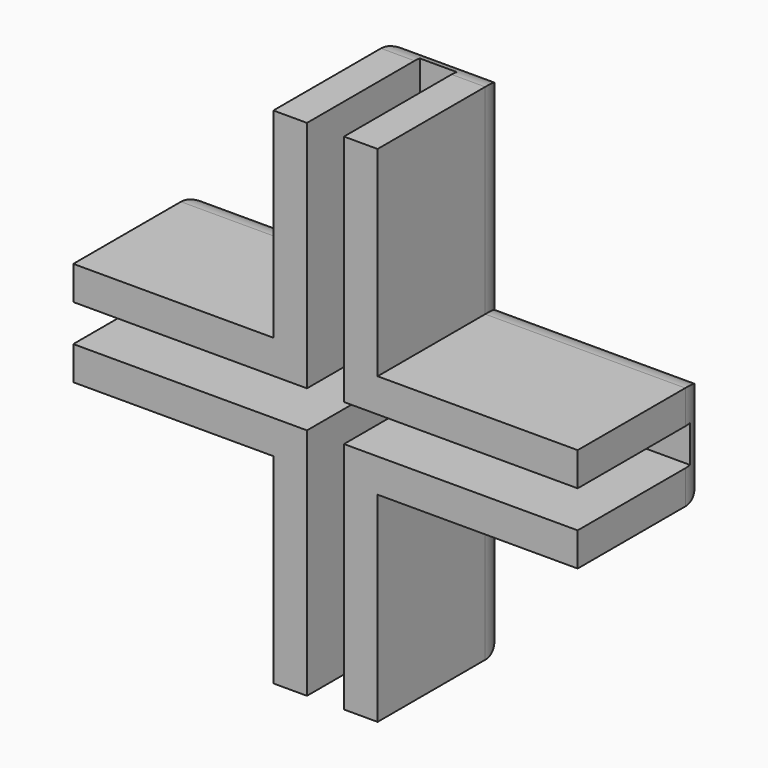
from build123d import *

# Parameters (mm, degrees)
F1_DEPTH     = 2.032
F2_DEPTH     = 12.7
F3_T1_DEPTH  = 21.463
F3_T3_DEPTH  = 21.463
F3_T5_DEPTH  = 20.574
F3_T7_DEPTH  = 21.463
F3_T9_DEPTH  = 20.574
F3_T11_DEPTH = 21.463
F3_T17_DEPTH = 27.813
F3_T21_DEPTH = 27.813
F3_T28_DEPTH = 27.813
F3_T32_DEPTH = 27.813
F3_T39_DEPTH = 27.813
F3_T43_DEPTH = 27.813
F3_T50_DEPTH = 27.813
F3_T54_DEPTH = 27.813


# Not quite as in the source:
# - a fillet or chamfer that OpenCascade refuses, or shapes differently, is made with other operations: its cross-section is extruded or revolved along the edge and cut away or added


with BuildPart() as f1:
    # F0 (on Front) → F1 (new body)
    with BuildSketch(Plane.XZ):
        Polygon((1.397, 19.05), (-1.397, 19.05), (-1.397, 1.397), (-19.05, 1.397), (-19.05, -1.397), (-1.397, -1.397), (-1.397, -19.05), (1.397, -19.05), (1.397, -1.397), (19.05, -1.397), (19.05, 1.397), (1.397, 1.397), align=None)
    extrude(amount=F1_DEPTH)

    # F0 (on Front) → F2 (join)
    with BuildSketch(Plane.XZ):
        Polygon((-1.397, 19.05), (-3.937, 19.05), (-3.937, 3.937), (-19.05, 3.937), (-19.05, 1.397), (-1.397, 1.397), align=None)
        Polygon((3.937, 19.05), (1.397, 19.05), (1.397, 1.397), (19.05, 1.397), (19.05, 3.937), (3.937, 3.937), align=None)
        Polygon((-1.397, -1.397), (-19.05, -1.397), (-19.05, -3.937), (-3.937, -3.937), (-3.937, -19.05), (-1.397, -19.05), align=None)
        Polygon((19.05, -3.937), (19.05, -1.397), (1.397, -1.397), (1.397, -19.05), (3.937, -19.05), (3.937, -3.937), align=None)
    extrude(amount=F2_DEPTH)

    # F3: fillet of radius 2.54 on 12 edges, made by hand

    # F3_s2 → F3_t1 (cut)
    with BuildSketch(Plane.XY.offset(3.937)):
        with BuildLine():
            ThreePointArc((-3.937, -2.54), (-3.1930512242, -0.7439487758), (-1.397, 0))
            Line((-1.397, 0), (-3.937, 0))
            Line((-3.937, 0), (-3.937, -2.54))
        make_face()
        with BuildLine():
            ThreePointArc((3.937, -2.54), (3.1930512242, -0.7439487758), (1.397, 0))
            Line((1.397, 0), (3.937, 0))
            Line((3.937, 0), (3.937, -2.54))
        make_face()
    extrude(amount=F3_T1_DEPTH, mode=Mode.SUBTRACT)

    # F3_s4 → F3_t3 (cut)
    with BuildSketch(Plane.YZ.offset(-25.4)):
        with BuildLine():
            ThreePointArc((-2.54, 3.937), (-0.7439487758, 3.1930512242), (0, 1.397))
            Line((0, 1.397), (0, 3.937))
            Line((0, 3.937), (-2.54, 3.937))
        make_face()
        with BuildLine():
            ThreePointArc((-2.54, -3.937), (-0.7439487758, -3.1930512242), (0, -1.397))
            Line((0, -1.397), (0, -3.937))
            Line((0, -3.937), (-2.54, -3.937))
        make_face()
    extrude(amount=F3_T3_DEPTH, mode=Mode.SUBTRACT)

    # F3_s6 → F3_t5 (cut)
    with BuildSketch(Plane.XY.offset(-10.287)):
        with BuildLine():
            ThreePointArc((-19.05, -2.54), (-18.3060512242, -0.7439487758), (-16.51, 0))
            Line((-16.51, 0), (-19.05, 0))
            Line((-19.05, 0), (-19.05, -2.54))
        make_face()
        with BuildLine():
            ThreePointArc((19.05, -2.54), (18.3060512242, -0.7439487758), (16.51, 0))
            Line((16.51, 0), (19.05, 0))
            Line((19.05, 0), (19.05, -2.54))
        make_face()
    extrude(amount=F3_T5_DEPTH, mode=Mode.SUBTRACT)

    # F3_s8 → F3_t7 (cut)
    with BuildSketch(Plane.XY.offset(-25.4)):
        with BuildLine():
            ThreePointArc((-3.937, -2.54), (-3.1930512242, -0.7439487758), (-1.397, 0))
            Line((-1.397, 0), (-3.937, 0))
            Line((-3.937, 0), (-3.937, -2.54))
        make_face()
        with BuildLine():
            ThreePointArc((3.937, -2.54), (3.1930512242, -0.7439487758), (1.397, 0))
            Line((1.397, 0), (3.937, 0))
            Line((3.937, 0), (3.937, -2.54))
        make_face()
    extrude(amount=F3_T7_DEPTH, mode=Mode.SUBTRACT)

    # F3_s10 → F3_t9 (cut)
    with BuildSketch(Plane.YZ.offset(-10.287)):
        with BuildLine():
            ThreePointArc((-2.54, -19.05), (-0.7439487758, -18.3060512242), (0, -16.51))
            Line((0, -16.51), (0, -19.05))
            Line((0, -19.05), (-2.54, -19.05))
        make_face()
        with BuildLine():
            ThreePointArc((-2.54, 19.05), (-0.7439487758, 18.3060512242), (0, 16.51))
            Line((0, 16.51), (0, 19.05))
            Line((0, 19.05), (-2.54, 19.05))
        make_face()
    extrude(amount=F3_T9_DEPTH, mode=Mode.SUBTRACT)

    # F3_s12 → F3_t11 (cut)
    with BuildSketch(Plane.YZ.offset(3.937)):
        with BuildLine():
            ThreePointArc((-2.54, -3.937), (-0.7439487758, -3.1930512242), (0, -1.397))
            Line((0, -1.397), (0, -3.937))
            Line((0, -3.937), (-2.54, -3.937))
        make_face()
        with BuildLine():
            ThreePointArc((-2.54, 3.937), (-0.7439487758, 3.1930512242), (0, 1.397))
            Line((0, 1.397), (0, 3.937))
            Line((0, 3.937), (-2.54, 3.937))
        make_face()
    extrude(amount=F3_T11_DEPTH, mode=Mode.SUBTRACT)


with BuildPart() as f3_tool15:
    # F3_s16 → F3_t17 (new body)
    with BuildSketch(Plane.XY.offset(25.4)):
        with BuildLine():
            ThreePointArc((-3.937, -2.54), (-3.1930512242, -0.7439487758), (-1.397, 0))
            Line((-1.397, 0), (-3.937, 0))
            Line((-3.937, 0), (-3.937, -2.54))
        make_face()
    extrude(amount=-F3_T17_DEPTH)

    split(bisect_by=Plane.XY.offset(3.937), keep=Keep.BOTTOM)


with BuildPart() as f3_tool19:
    # F3_s20 → F3_t21 (new body)
    with BuildSketch(Plane.YZ.offset(2.413)):
        with BuildLine():
            ThreePointArc((-2.54, 3.937), (-0.7439487758, 3.1930512242), (0, 1.397))
            Line((0, 1.397), (0, 3.937))
            Line((0, 3.937), (-2.54, 3.937))
        make_face()
    extrude(amount=-F3_T21_DEPTH)

    split(bisect_by=Plane.YZ.offset(-3.937), keep=Keep.TOP)


with BuildPart() as f3_tool15_1:
    add(f3_tool15.part)

    # F3_t23: intersect F3_tool19
    add(f3_tool19.part, mode=Mode.INTERSECT)


with BuildPart() as f1_1:
    add(f1.part)

    # F3_t13: cut F3_tool15
    add(f3_tool15_1.part, mode=Mode.SUBTRACT)


with BuildPart() as f3_tool26:
    # F3_s27 → F3_t28 (new body)
    with BuildSketch(Plane.YZ.offset(-25.4)):
        with BuildLine():
            ThreePointArc((-2.54, -3.937), (-0.7439487758, -3.1930512242), (0, -1.397))
            Line((0, -1.397), (0, -3.937))
            Line((0, -3.937), (-2.54, -3.937))
        make_face()
    extrude(amount=F3_T28_DEPTH)

    split(bisect_by=Plane.YZ.offset(-3.937), keep=Keep.TOP)


with BuildPart() as f3_tool30:
    # F3_s31 → F3_t32 (new body)
    with BuildSketch(Plane.XY.offset(2.413)):
        with BuildLine():
            ThreePointArc((-3.937, -2.54), (-3.1930512242, -0.7439487758), (-1.397, 0))
            Line((-1.397, 0), (-3.937, 0))
            Line((-3.937, 0), (-3.937, -2.54))
        make_face()
    extrude(amount=-F3_T32_DEPTH)

    split(bisect_by=Plane.XY.offset(-3.937), keep=Keep.TOP)


with BuildPart() as f3_tool26_1:
    add(f3_tool26.part)

    # F3_t34: intersect F3_tool30
    add(f3_tool30.part, mode=Mode.INTERSECT)


with BuildPart() as f1_2:
    add(f1_1.part)

    # F3_t24: cut F3_tool26
    add(f3_tool26_1.part, mode=Mode.SUBTRACT)


with BuildPart() as f3_tool37:
    # F3_s38 → F3_t39 (new body)
    with BuildSketch(Plane.XY.offset(-25.4)):
        with BuildLine():
            ThreePointArc((3.937, -2.54), (3.1930512242, -0.7439487758), (1.397, 0))
            Line((1.397, 0), (3.937, 0))
            Line((3.937, 0), (3.937, -2.54))
        make_face()
    extrude(amount=F3_T39_DEPTH)

    split(bisect_by=Plane.XY.offset(-3.937), keep=Keep.TOP)


with BuildPart() as f3_tool41:
    # F3_s42 → F3_t43 (new body)
    with BuildSketch(Plane.YZ.offset(-2.413)):
        with BuildLine():
            ThreePointArc((-2.54, -3.937), (-0.7439487758, -3.1930512242), (0, -1.397))
            Line((0, -1.397), (0, -3.937))
            Line((0, -3.937), (-2.54, -3.937))
        make_face()
    extrude(amount=F3_T43_DEPTH)

    split(bisect_by=Plane.YZ.offset(3.937), keep=Keep.BOTTOM)


with BuildPart() as f3_tool37_1:
    add(f3_tool37.part)

    # F3_t45: intersect F3_tool41
    add(f3_tool41.part, mode=Mode.INTERSECT)


with BuildPart() as f1_3:
    add(f1_2.part)

    # F3_t35: cut F3_tool37
    add(f3_tool37_1.part, mode=Mode.SUBTRACT)


with BuildPart() as f3_tool48:
    # F3_s49 → F3_t50 (new body)
    with BuildSketch(Plane.YZ.offset(25.4)):
        with BuildLine():
            ThreePointArc((-2.54, 3.937), (-0.7439487758, 3.1930512242), (0, 1.397))
            Line((0, 1.397), (0, 3.937))
            Line((0, 3.937), (-2.54, 3.937))
        make_face()
    extrude(amount=-F3_T50_DEPTH)

    split(bisect_by=Plane.YZ.offset(3.937), keep=Keep.BOTTOM)


with BuildPart() as f3_tool52:
    # F3_s53 → F3_t54 (new body)
    with BuildSketch(Plane.XY.offset(-2.413)):
        with BuildLine():
            ThreePointArc((3.937, -2.54), (3.1930512242, -0.7439487758), (1.397, 0))
            Line((1.397, 0), (3.937, 0))
            Line((3.937, 0), (3.937, -2.54))
        make_face()
    extrude(amount=F3_T54_DEPTH)

    split(bisect_by=Plane.XY.offset(3.937), keep=Keep.BOTTOM)


with BuildPart() as f3_tool48_1:
    add(f3_tool48.part)

    # F3_t56: intersect F3_tool52
    add(f3_tool52.part, mode=Mode.INTERSECT)


with BuildPart() as f1_4:
    add(f1_3.part)

    # F3_t46: cut F3_tool48
    add(f3_tool48_1.part, mode=Mode.SUBTRACT)


solid = f1_4.part
